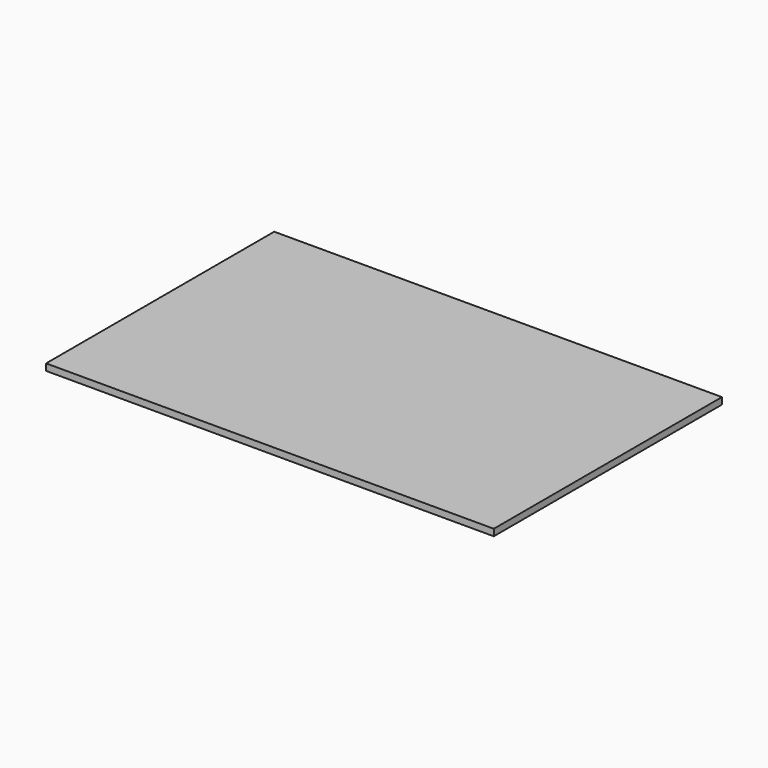
from build123d import *

# Parameters (mm, degrees)
F0_W     = 1066.8
F0_H     = 679.45
F1_DEPTH = 15.875


# Not quite as in the source:
# - a length typed as a fraction of an inch, garbled in the dataset ("3 / 203.2 mm" for 3/8 in), is restored


with BuildPart() as f1:
    # F0 (on Top) → F1 (new body)
    with BuildSketch(Plane.XY):
        with Locations((533.4, 339.725)):
            Rectangle(F0_W, F0_H)
    extrude(amount=F1_DEPTH)


solid = f1.part
